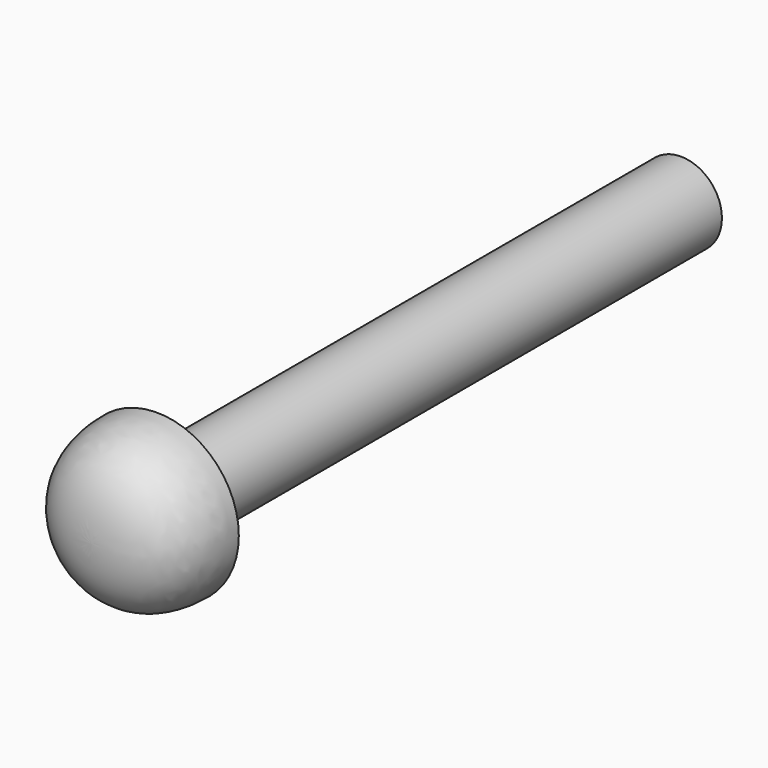
from build123d import *

# Parameters (mm, degrees)
F0_R     = 6.35
F1_DEPTH = 101.5999987721
F2_R     = 12.7
F3_DEPTH = 12.7


# Not quite as in the source:
# - a fillet or chamfer that OpenCascade refuses, or shapes differently, is made with other operations: its cross-section is extruded or revolved along the edge and cut away or added


with BuildPart() as f1:
    # F0 (on Front) → F1 (new body)
    with BuildSketch(Plane.XZ):
        Circle(F0_R)
    extrude(amount=-F1_DEPTH)

    # F2 (on face) + F0 (on Front) → F3 (join)
    with BuildSketch(Plane.XZ):
        Circle(F2_R)
    with BuildSketch(Plane.XZ):
        Circle(F0_R)
    extrude(amount=F3_DEPTH)

    # F4: fillet of radius 12.7 on 1 edges, made by hand

    # F4_s1 → F4_t2 (revolve, cut)
    with BuildSketch(Plane.XY):
        with BuildLine():
            add(Edge.make_bspline(
                [(12.7, 0), (12.7, -12.7), (0, -12.7)],
                knots=[0, 0, 0, 1, 1, 1], degree=2, weights=[1, 1, 1]))
            Line((0, -12.7), (12.7, -12.7))
            Line((12.7, -12.7), (12.7, 0))
        make_face()
    revolve(axis=Axis((0, -12.7, 0), (0, -1, 0)), mode=Mode.SUBTRACT)


solid = f1.part
